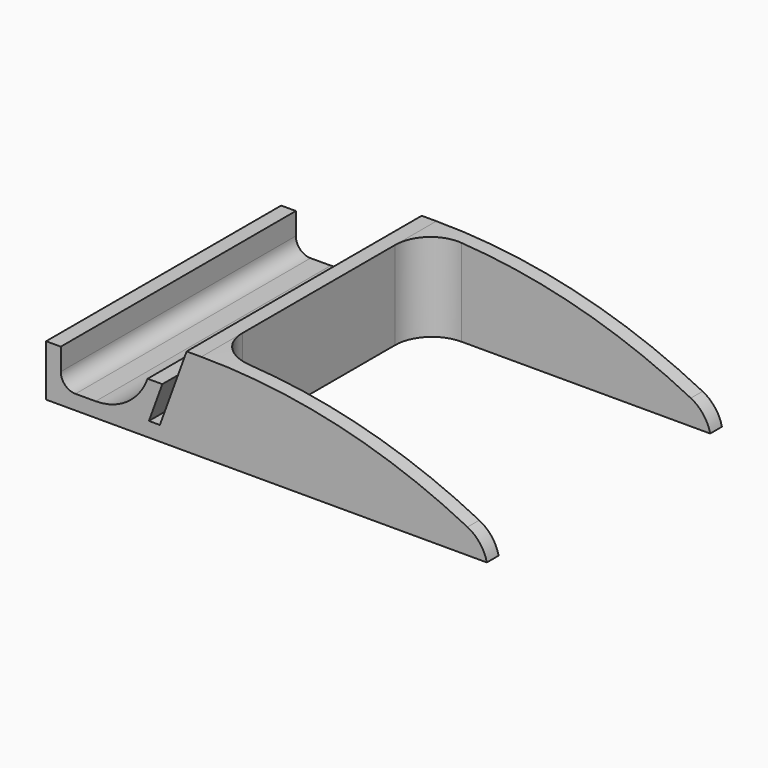
from build123d import *

# Parameters (mm, degrees)
F1_DEPTH    = 40
F2_W        = 38.8704487759
F2_H        = 36
F3_DEPTH    = 25
F4_R        = 7.5
F5_R        = 2
F6_T1_DEPTH = 16.8824680596
F6_T3_DEPTH = 16.8824680596
F7_R        = 5


# Not quite as in the source:
# - a fillet or chamfer that OpenCascade refuses, or shapes differently, is made with other operations: its cross-section is extruded or revolved along the edge and cut away or added


with BuildPart() as f1:
    # F0 (on Front) → F1 (new body)
    with BuildSketch(Plane.XZ):
        with BuildLine():
            Line((0, -2), (0, 0))
            ThreePointArc((0, 0), (-18.8023659823, 7.4599490238), (-38.8704487759, 10))
            Line((-38.8704487759, 10), (-40.8704487759, 10))
            Line((-40.8704487759, 10), (-44.5101511185, 0))
            Line((-44.5101511185, 0), (-46, 0))
            Line((-46, 0), (-44.1801488287, 5))
            Line((-44.1801488287, 5), (-46.1801488287, 5))
            Line((-46.1801488287, 5), (-48, 0))
            Line((-48, 0), (-58, 0))
            Line((-58, 0), (-58, 5))
            Line((-58, 5), (-60, 5))
            Line((-60, 5), (-60, -2))
            Line((-60, -2), (0, -2))
        make_face()
    extrude(amount=F1_DEPTH)

    # F2 (on face) → F3 (cut)
    with BuildSketch(Plane.XY.offset(10)):
        with Locations((-19.4352243879, -20)):
            Rectangle(F2_W, F2_H)
    extrude(amount=-F3_DEPTH, mode=Mode.SUBTRACT)

    # F4
    f4_edges = [f1.edges().sort_by_distance(p)[0] for p in [
        (-48, -20, 0),
    ]]
    fillet(f4_edges, radius=F4_R)

    # F5
    f5_edges = [f1.edges().sort_by_distance(p)[0] for p in [
        (-58, -20, 0),
    ]]
    fillet(f5_edges, radius=F5_R)

    # F6: fillet of radius 5 on 2 edges, made by hand

    # F6_s2 → F6_t1 (cut)
    with BuildSketch(Plane.XZ.offset(30.5587659702)):
        with BuildLine():
            ThreePointArc((0, -2), (-0.9346139409, -0.0091871804), (-2.6330480047, 1.3880102401))
            ThreePointArc((-2.6330480047, 1.3880102401), (-1.3101118631, 0.7061689139), (0, 0))
            Line((0, 0), (0, -2))
        make_face()
    extrude(amount=F6_T1_DEPTH, mode=Mode.SUBTRACT)

    # F6_s4 → F6_t3 (cut)
    with BuildSketch(Plane.XZ.offset(-7.4412340298)):
        with BuildLine():
            ThreePointArc((0, -2), (-0.9346139409, -0.0091871804), (-2.6330480047, 1.3880102401))
            ThreePointArc((-2.6330480047, 1.3880102401), (-1.3101118631, 0.7061689139), (0, 0))
            Line((0, 0), (0, -2))
        make_face()
    extrude(amount=F6_T3_DEPTH, mode=Mode.SUBTRACT)

    # F7
    f7_edges = [f1.edges().sort_by_distance(p)[0] for p in [
        (-38.870449, -38, 4),
        (-38.870449, -2, 4),
    ]]
    fillet(f7_edges, radius=F7_R)


solid = f1.part
